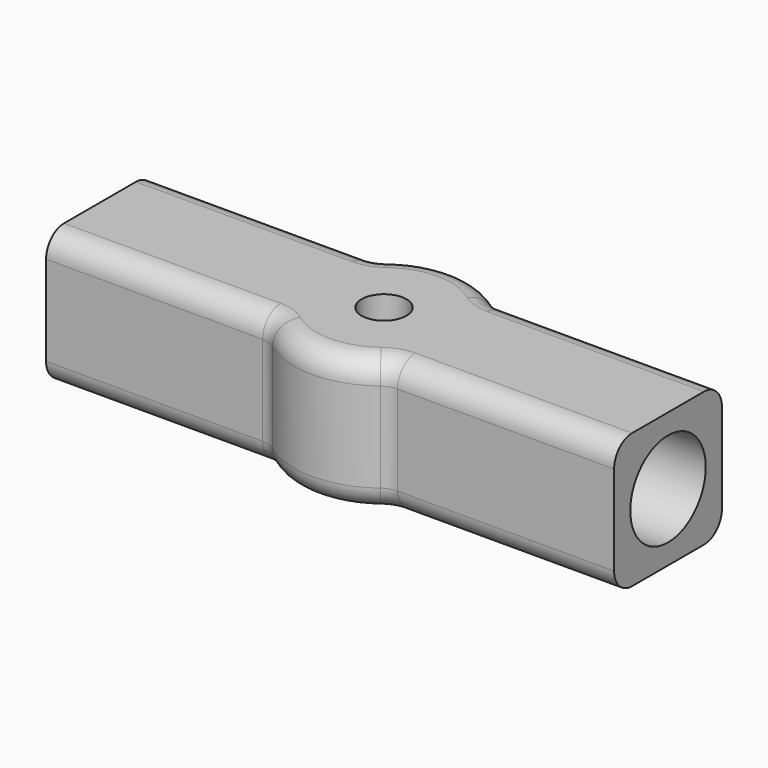
from build123d import *

# Parameters (mm, degrees)
F0_R     = 1
F1_DEPTH = 6
F2_R     = 2.1
F3_DEPTH = 10
F4_F1_R  = 1
F4_F2_R  = 1


with BuildPart() as f1:
    # F0 (on Top) → F1 (new body)
    with BuildSketch(Plane.XY):
        with BuildLine():
            Line((12.645751, 3), (2.645751, 3))
            ThreePointArc((2.645751, 3), (-4, 0), (2.645751, -3))
            Line((2.645751, -3), (12.645751, -3))
            Line((12.645751, -3), (12.645751, 3))
        make_face()
        Circle(F0_R, mode=Mode.SUBTRACT)
    extrude(amount=F1_DEPTH)

    # F2 (on face) → F3 (cut)
    with BuildSketch(Plane.YZ.offset(12.645751)):
        with Locations((0, 3)):
            Circle(F2_R)
    extrude(amount=-F3_DEPTH, mode=Mode.SUBTRACT)

    # F4: fillet of radius 1 on 4 edges, made by hand

    # F4_f1
    f4_f1_edges = [f1.edges().sort_by_distance(p)[0] for p in [
        (2.645751, 3, 3),
        (2.645751, -3, 3),
    ]]
    fillet(f4_f1_edges, radius=F4_F1_R)

    # F4_f2
    f4_f2_edges = [f1.edges().sort_by_distance(p)[0] for p in [
        (7.822876, -3, 6),
        (7.822876, -3, 0),
        (2.683772, -3.051317, 0),
        (2.683772, -3.051317, 6),
    ]]
    fillet(f4_f2_edges, radius=F4_F2_R)

    # F5: F1 across plane


with BuildPart() as f1_1:
    add(f1.part)
    add(f1.part.mirror(Plane.YZ))


solid = f1_1.part
